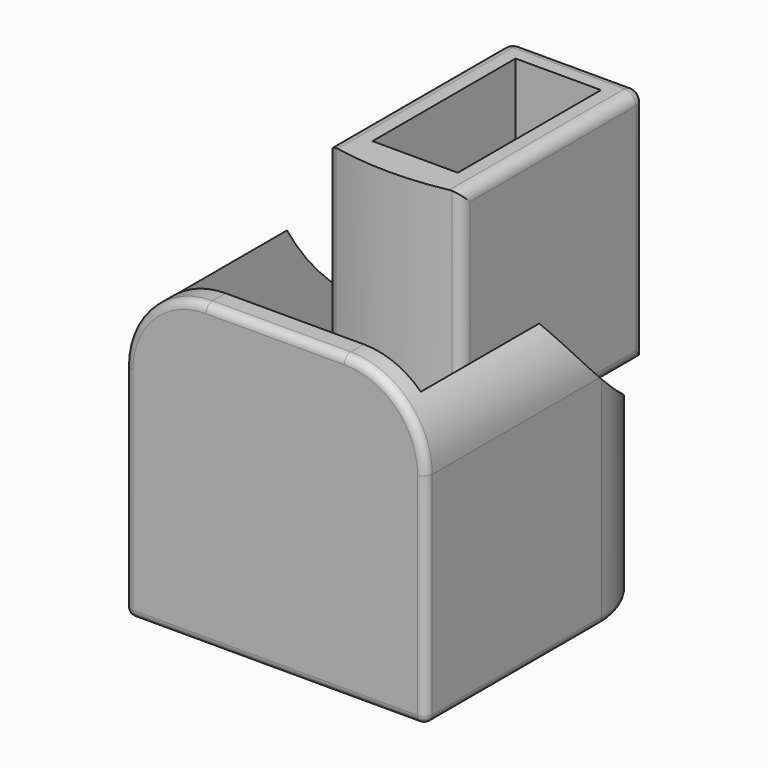
from build123d import *

# Parameters (mm, degrees)
F0_W         = 18.5
F0_H         = 18.5
F1_DEPTH     = 18.5
F2_R         = 19
F3_DEPTH     = 25.4
F4_T         = -1.5
F6_DEPTH     = 14
F7_T         = 1.5
F7_T3_DEPTH  = 3.8130317325
F7_T5_DEPTH  = 20
F7_T7_DEPTH  = 18.5
F7_T9_DEPTH  = 12.1348502244
F7_T11_DEPTH = 18.5
F7_T13_DEPTH = 4.6348502244
F7_T16_ANGLE = 5.1594967302
F7_T18_ANGLE = 27.6449084771
F7_T20_ANGLE = 5.1594967302
F7_T22_ANGLE = 27.6449084771
F9_DEPTH     = 23.32034
F10_DEPTH    = 8.55107
F11_R        = 5
F12_R        = 0.7
F13_R        = 0.5


# Not quite as in the source:
# - a shell that OpenCascade refuses in one call is made with other operations: the cavity is built on its own and cut out


with BuildPart() as f1:
    # F0 (on Top) → F1 (new body)
    with BuildSketch(Plane.XY):
        Rectangle(F0_W, F0_H)
    extrude(amount=-F1_DEPTH)

    # F2 (on face) → F3 (cut)
    with BuildSketch(Plane.YZ.offset(9.25)):
        with Locations((17.6200576851, 8.3700576851)):
            Circle(F2_R)
    extrude(amount=-F3_DEPTH, mode=Mode.SUBTRACT)

    # F4
    f4_openings = [f1.faces().sort_by_distance(p)[0] for p in [
        (0, -4.343484, 0),
        (0, 4.185029, -5.064971),
    ]]
    offset(amount=F4_T, openings=f4_openings)

    # F5 (on Front) → F6 (join)
    with BuildSketch(Plane.XZ):
        with BuildLine():
            Line((4.125, -9.5), (4.125, 5))
            Line((4.125, 5), (0, 5))
            Line((0, 5), (-4.125, 5))
            Line((-4.125, 5), (-4.125, -9.5))
            ThreePointArc((-4.125, -9.5), (0, -10), (4.125, -9.5))
        make_face()
    extrude(amount=-F6_DEPTH)

    # F7: shell of thickness 1.5, made by hand


with BuildPart() as f7_core1:
    # F7_t2: copy of F1
    add(f1.part)

    # the walls: a layer under each face that stays
    f7_faces = [f7_core1.faces().sort_by_distance(p)[0] for p in [
        (9.25, 0, -9.25),
        (-7.9285714286, -8.549069162, 0),
        (8.3958333333, 1.5822898542, -1.8176801895),
        (0, 9.25, -13.5934841338),
        (0, 0, -18.5),
        (0, -9.25, -9.25),
        (-8.3958333333, 1.5822898542, -1.8176801895),
        (-9.25, 0, -9.25),
        (7.75, 0, -8.5),
        (0, -7.75, -8.5),
        (-7.75, 0, -8.5),
        (4.125, 7, -2.25),
        (0, 7.75, -12.4325748878),
        (0, 11.625, -10),
        (-4.125, 7, -2.25),
        (0, 0, -17),
        (0, 0, -2.5),
        (0, 14, -2.5),
        (0, 3.875, -10),
    ]]
    thicken(f7_faces, amount=-F7_T, mode=Mode.SUBTRACT)

    # F7_s4 → F7_t3 (cut)
    with BuildSketch(Plane.XY.offset(-11)):
        Polygon((4.14, 9.265), (4.125, 7.75), (2.625, 7.75), (2.625, 9.25), align=None)
        Polygon((-4.14, 9.265), (-4.125, 7.75), (-2.625, 7.75), (-2.625, 9.25), align=None)
    extrude(amount=F7_T3_DEPTH, mode=Mode.SUBTRACT)

    # F7_s6 → F7_t5 (cut)
    with BuildSketch(Plane.XY.offset(-18.5)):
        Polygon((7.735, -7.735), (9.25, -7.75), (9.25, -9.25), (7.75, -9.25), align=None)
        Polygon((-7.735, -7.735), (-7.75, -9.25), (-9.25, -9.25), (-9.25, -7.75), align=None)
    extrude(amount=F7_T5_DEPTH, mode=Mode.SUBTRACT)

    # F7_s8 → F7_t7 (cut)
    with BuildSketch(Plane.XZ.offset(-9.25)):
        Polygon((7.735, -16.985), (9.25, -17), (9.25, -18.5), (7.75, -18.5), align=None)
        Polygon((-7.735, -16.985), (-9.25, -17), (-9.25, -18.5), (-7.75, -18.5), align=None)
    extrude(amount=F7_T7_DEPTH, mode=Mode.SUBTRACT)

    # F7_s10 → F7_t9 (cut)
    with BuildSketch(Plane.XY.offset(-18.5)):
        Polygon((7.735, 7.735), (9.25, 7.75), (9.25, 9.25), (7.75, 9.25), align=None)
        Polygon((-7.735, 7.735), (-9.25, 7.75), (-9.25, 9.25), (-7.75, 9.25), align=None)
    extrude(amount=F7_T9_DEPTH, mode=Mode.SUBTRACT)

    # F7_s12 → F7_t11 (cut)
    with BuildSketch(Plane.YZ.offset(-9.25)):
        Polygon((-7.735, -16.985), (-9.25, -17), (-9.25, -18.5), (-7.75, -18.5), align=None)
        Polygon((7.735, -16.985), (9.25, -17), (9.25, -18.5), (7.75, -18.5), align=None)
    extrude(amount=F7_T11_DEPTH, mode=Mode.SUBTRACT)

    # F7_s14 → F7_t13 (cut)
    with BuildSketch(Plane.XY.offset(-11)):
        Polygon((4.14, 7.735), (2.625, 7.75), (2.625, 9.25), (4.125, 9.25), align=None)
        Polygon((-4.14, 7.735), (-4.125, 9.25), (-2.625, 9.25), (-2.625, 7.75), align=None)
    extrude(amount=F7_T13_DEPTH, mode=Mode.SUBTRACT)

    # F7_s15 → F7_t16 (revolve, cut)
    with BuildSketch(Plane(origin=(0, 9.1498364132, -5.5625660113), x_dir=(1, 0, 0), z_dir=(0, -0.8544846032, 0.5194767203))):
        Polygon((4.14, -2.679704803), (4.125, -4.194704803), (2.625, -4.194704803), (2.625, -2.694704803), align=None)
    revolve(axis=Axis((4.125, 17.6200576851, 8.3700576851), (1, 0, 0)), revolution_arc=F7_T16_ANGLE, mode=Mode.SUBTRACT)

    # F7_s17 → F7_t18 (revolve, cut)
    with BuildSketch(Plane(origin=(-1.6855904875, 0, 0.4147212383), x_dir=(0, 1, 0), z_dir=(-0.971040724, 0, 0.2389140271))):
        Polygon((9.265, 10.2254072398), (7.75, 10.2104072398), (7.75, 8.7104072398), (9.25, 8.7104072398), align=None)
    revolve(axis=Axis((0, 9.25, 7.265625), (0, -1, 0)), revolution_arc=F7_T18_ANGLE, mode=Mode.SUBTRACT)

    # F7_s19 → F7_t20 (revolve, cut)
    with BuildSketch(Plane(origin=(0, 9.1498364132, -5.5625660113), x_dir=(1, 0, 0), z_dir=(0, -0.8544846032, 0.5194767203))):
        Polygon((-4.14, -2.679704803), (-4.125, -4.194704803), (-2.625, -4.194704803), (-2.625, -2.694704803), align=None)
    revolve(axis=Axis((-4.125, 17.6200576851, 8.3700576851), (1, 0, 0)), revolution_arc=F7_T20_ANGLE, mode=Mode.SUBTRACT)

    # F7_s21 → F7_t22 (revolve, cut)
    with BuildSketch(Plane(origin=(-1.6855904875, 0, 0.4147212383), x_dir=(0, 1, 0), z_dir=(-0.971040724, 0, 0.2389140271))):
        Polygon((7.735, 10.2254072398), (9.25, 10.2104072398), (9.25, 8.7104072398), (7.75, 8.7104072398), align=None)
    revolve(axis=Axis((0, 7.75, 7.265625), (0, -1, 0)), revolution_arc=F7_T22_ANGLE, mode=Mode.SUBTRACT)


with BuildPart() as f1_1:
    add(f1.part)

    # what is left inside the walls is the cavity
    f7_cavity = [f7_core1.part.solids().sort_by_distance(p)[0] for p in [
        (-2.61, 7, 0.573356),
    ]]
    add(f7_cavity, mode=Mode.SUBTRACT)

    # F8 (on face) → F9 (join)
    with BuildSketch(Plane.XY.offset(5)):
        with BuildLine():
            Line((4.125, 0), (-4.125, 0))
            ThreePointArc((-4.125, 0), (0, -0.5), (4.125, 0))
        make_face()
    extrude(amount=-F9_DEPTH)

    # F10 (add): a face of the model
    f10_faces = [f1_1.faces().sort_by_distance(p)[0] for p in [
        (0, 0, -13.4156113664),
    ]]
    extrude(f10_faces, amount=F10_DEPTH)

    # F11
    f11_edges = [f1_1.edges().sort_by_distance(p)[0] for p in [
        (-9.25, -4.343484, 0),
        (9.25, -4.343484, 0),
        (9.25, 9.25, -13.593484),
        (-9.25, 9.25, -13.593484),
    ]]
    fillet(f11_edges, radius=F11_R)

    # F12
    f12_edges = [f1_1.edges().sort_by_distance(p)[0] for p in [
        (4.125, 14, -2.25),
        (-4.125, 14, -2.25),
        (4.125, 7, 5),
        (-4.125, 7, 5),
        (-4.125, 11.625, -9.5),
        (4.125, 11.625, -9.5),
        (4.125, 0, -6),
        (-4.125, 0, -6),
        (0, 14, 5),
    ]]
    fillet(f12_edges, radius=F12_R)

    # F13
    f13_edges = [f1_1.edges().sort_by_distance(p)[0] for p in [
        (9.25, -2.5, -18.5),
        (0, -9.25, -18.5),
        (9.25, -9.25, -11.75),
        (-9.25, -2.5, -18.5),
        (-9.25, -9.25, -11.75),
        (0, 9.25, -18.5),
        (7.785534, 7.785534, -18.5),
        (-7.785534, 7.785534, -18.5),
        (7.785534, -9.25, -1.464466),
        (-7.785534, -9.25, -1.464466),
        (0, -9.25, 0),
    ]]
    fillet(f13_edges, radius=F13_R)


solid = f1_1.part
